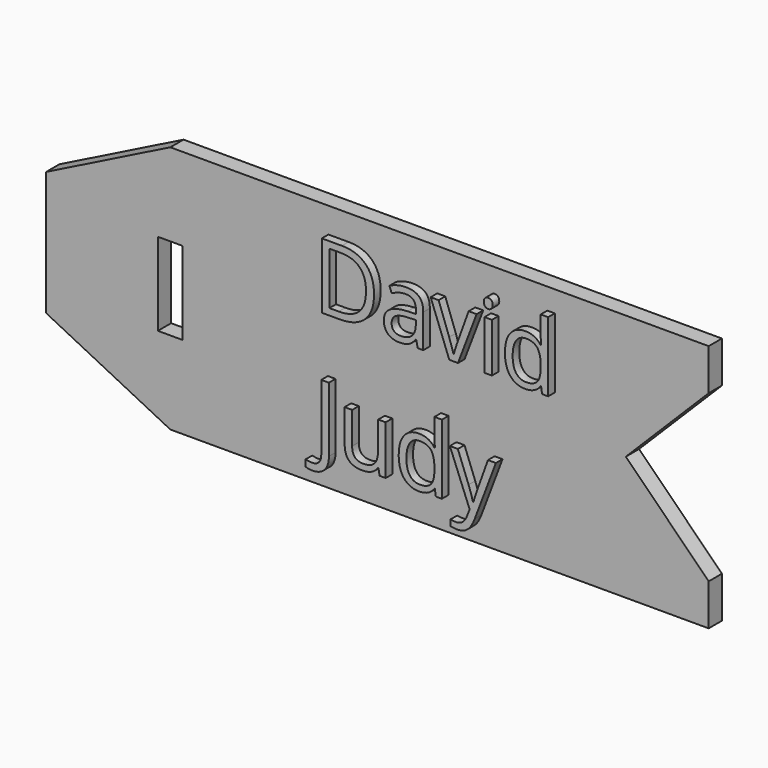
from build123d import *

# Parameters (mm, degrees)
F0_W         = 3
F0_H         = 10
F1_DEPTH     = 2
F2_TEXT_SIZE = 11.0745803772
F3_DEPTH     = 1


# Not quite as in the source:
# - Text() gives the source's letters only with a copy of the font that has no kerning and outlines rounded to 1/6400 em; it was checked with that copy


with BuildPart() as f1:
    # F0 (on Front) → F1 (new body)
    with BuildSketch(Plane.XZ):
        Polygon((-25, -15), (40, -15), (40, -10), (30, 0), (40, 10), (40, 15), (-25, 15), (-40, 7.5), (-40, -7.5), align=None)
        with Locations((-25, 0)):
            Rectangle(F0_W, F0_H, mode=Mode.SUBTRACT)
    extrude(amount=F1_DEPTH)

    # F2 (on face) → F3 (join)
    with BuildSketch(Plane.XZ.offset(2)):
        with Locations((-7, 4.0263021284)):
            Text('David', F2_TEXT_SIZE, font='Open Sans', text_align=(TextAlign.LEFT, TextAlign.BOTTOM))
        with Locations((-7, -11.0351271846)):
            Text('Judy', F2_TEXT_SIZE, font='Open Sans', text_align=(TextAlign.LEFT, TextAlign.BOTTOM))
    extrude(amount=F3_DEPTH)


solid = f1.part
